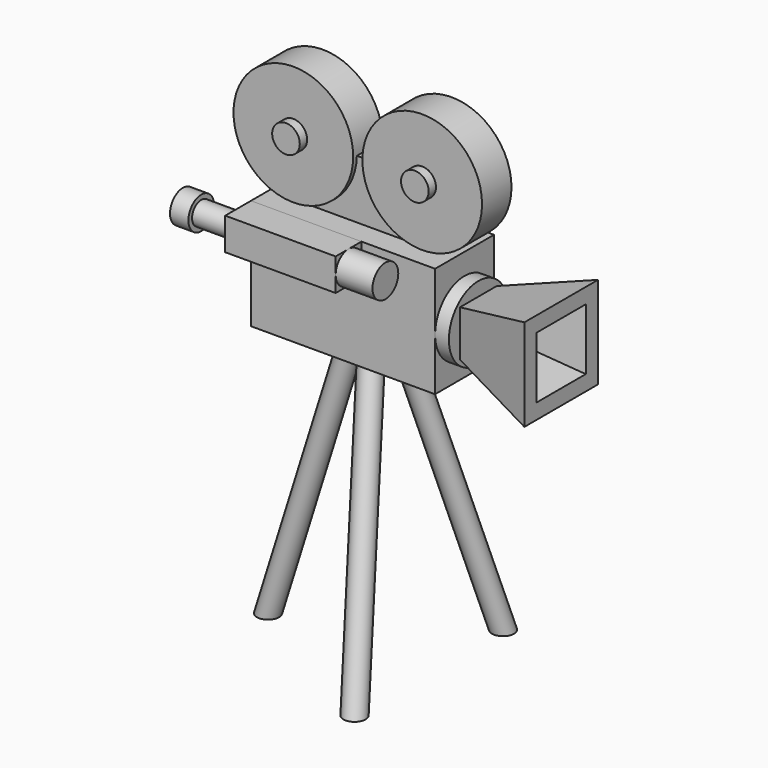
from build123d import *

# Parameters (mm, degrees)
F0_W      = 10
F0_H      = 6
F1_DEPTH  = 2
F2_R      = 3.25
F3_DEPTH  = 1
F5_DEPTH  = 0.75
F6_R      = 0.75
F7_DEPTH  = 1.5
F8_R      = 2
F9_DEPTH  = 0.75
F12_W     = 5
F12_H     = 5
F10_W     = 2.5
F10_H     = 2.5
F14_T     = -0.8
F15_W     = 1.75
F15_H     = 1.75
F16_DEPTH = 6
F17_R     = 0.875
F18_DEPTH = 2
F19_R     = 0.625
F20_DEPTH = 3
F21_R     = 0.875
F22_DEPTH = 1
F25_R     = 0.6
F29_COUNT = 3
F29_ANGLE = 240


# Not quite as in the source:
# - the program builds the solid bodies; features that only make, move or delete a surface that nothing else refers to are left out


with BuildPart() as f1:
    # F0 (on Front) → F1 (new body, symmetric)
    with BuildSketch(Plane.XZ):
        with Locations((-0.1466497779, 0.1515977762)):
            Rectangle(F0_W, F0_H)
    extrude(amount=F1_DEPTH, both=True)

    # F8 (on face) → F9 (join)
    with BuildSketch(Plane.YZ.offset(4.8533502221)):
        Circle(F8_R)
    extrude(amount=F9_DEPTH)

    # F12 (on offset) → F13 section 0
    with BuildSketch(Plane.YZ.offset(10.1033502221)):
        Rectangle(F12_W, F12_H)
    # F10 (on face) → F13 section 1
    with BuildSketch(Plane.YZ.offset(5.6033502221)):
        Rectangle(F10_W, F10_H)
    loft()

    # F14
    f14_openings = [f1.faces().sort_by_distance(p)[0] for p in [
        (10.10335, 0, 0),
    ]]
    offset(amount=F14_T, openings=f14_openings, kind=Kind.INTERSECTION)


with BuildPart() as f3:
    # F2 (on Front) → F3 (new body, symmetric)
    with BuildSketch(Plane.XZ):
        with Locations((-3.6466497779, 6.4015977762)):
            Circle(F2_R)
    extrude(amount=F3_DEPTH, both=True)


with BuildPart() as f3b:
    # F2 (on Front) → F3, piece 2 (new body, symmetric)
    with BuildSketch(Plane.XZ):
        with Locations((3.3533502221, 6.4015977762)):
            Circle(F2_R)
    extrude(amount=F3_DEPTH, both=True)


with BuildPart() as f5:
    # F4 (on Front) → F5 (new body, symmetric)
    with BuildSketch(Plane.XZ):
        with BuildLine():
            ThreePointArc((-0.3972530839, 6.3389788862), (-1.3707995403, 4.0814672419), (-3.6466497779, 3.1515977762))
            Line((-3.6466497779, 3.1515977762), (3.3533502221, 3.1515977762))
            ThreePointArc((3.3533502221, 3.1515977762), (1.0774999845, 4.0814672419), (0.1039535282, 6.3389788862))
            Line((0.1039535282, 6.3389788862), (-0.3972530839, 6.3389788862))
        make_face()
    extrude(amount=F5_DEPTH, both=True)


with BuildPart() as f7:
    # F6 (on Front) → F7 (new body, symmetric)
    with BuildSketch(Plane.XZ):
        with Locations((-3.6466497779, 6.4015977762)):
            Circle(F6_R)
    extrude(amount=F7_DEPTH, both=True)


with BuildPart() as f7b:
    # F6 (on Front) → F7, piece 2 (new body, symmetric)
    with BuildSketch(Plane.XZ):
        with Locations((3.3533502221, 6.4015977762)):
            Circle(F6_R)
    extrude(amount=F7_DEPTH, both=True)


with BuildPart() as f16:
    # F15 (on face) → F16 (new body)
    with BuildSketch(Plane(origin=(-5.1466497779, 0, 0), x_dir=(0, -1, 0), z_dir=(-1, 0, 0))):
        with Locations((2.875, 2.2765977762)):
            Rectangle(F15_W, F15_H)
    extrude(amount=-F16_DEPTH)

    # F19 (on face) → F20 (join)
    with BuildSketch(Plane(origin=(-5.1466497779, 0, 0), x_dir=(0, -1, 0), z_dir=(-1, 0, 0))):
        with Locations((2.875, 2.2765977762)):
            Circle(F19_R)
    extrude(amount=F20_DEPTH)

    # F21 (on face) → F22 (join)
    with BuildSketch(Plane(origin=(-8.1466497779, 0, 0), x_dir=(0, -1, 0), z_dir=(-1, 0, 0))):
        with Locations((2.875, 2.2765977762)):
            Circle(F21_R)
    extrude(amount=-F22_DEPTH)


with BuildPart() as f18:
    # F17 (on face) → F18 (new body)
    with BuildSketch(Plane.YZ.offset(0.8533502221)):
        with Locations((-2.875, 2.2765977762)):
            Circle(F17_R)
    extrude(amount=F18_DEPTH)


with BuildPart() as f27:
    # F27: sweep along a path in F26
    with BuildLine(Plane.XZ) as f27_path:
        Line((-1.2, -2.8484022238), (-5.8201700449, -17.6013689488))
    # F25 (on face) → F27 (sweep)
    with BuildSketch(Plane(origin=(0, 0, -2.8484022238), x_dir=(1, 0, 0), z_dir=(0, 0, -1))):
        with Locations((-1.2, 0)):
            Circle(F25_R)
    sweep(path=f27_path.line)


with BuildPart() as f29_1:
    # F29: instance of F27
    add(f27.part.rotate(Axis((0, 0, 0.4013092257), (0, 0, -1)), 1 * F29_ANGLE / (F29_COUNT - 1)))


with BuildPart() as f29_2:
    # F29: instance of F27
    add(f27.part.rotate(Axis((0, 0, 0.4013092257), (0, 0, -1)), 2 * F29_ANGLE / (F29_COUNT - 1)))


solid = Compound([f1.part, f3.part, f3b.part, f5.part, f7.part, f7b.part, f16.part, f18.part, f27.part, f29_1.part, f29_2.part])
